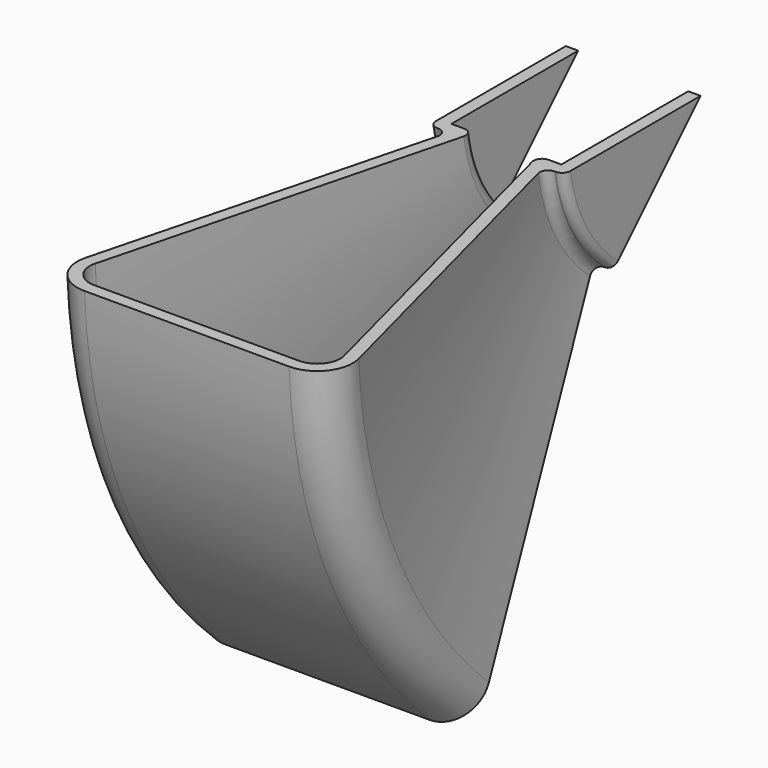
from build123d import *

# Parameters (mm, degrees)
F1_ANGLE_BACK  = 30
F1_ANGLE       = 120
F2_R           = 2
F4_DEPTH       = 25
F4_DEPTH_BACK  = 25
F5_DEPTH       = 25
F5_DEPTH_BACK  = 25
F8_R           = 5
F10_DEPTH      = 33.4248144675
F10_DEPTH_BACK = 33.4248144675
F12_DEPTH      = 50
F12_DEPTH_BACK = 50


# Not quite as in the source:
# - after a boolean that leaves OpenCascade's solid faulty, fix() repairs it
# - a feature of the source that left no trace in its solid (it failed there, or was rolled back) is left out


with BuildPart() as f1:
    # F0 (on Top) → F1 (revolve)
    with BuildSketch(Plane.XY, mode=Mode.PRIVATE) as f1_sk:
        with BuildLine():
            Line((9.6206148389, -1.9516889929), (7.6821408379, -2.0284350604))
            Line((7.6821408379, -2.0284350604), (30.2427770644, -88.5876107865))
            ThreePointArc((30.2427770644, -88.5876107865), (29.2549191731, -93.4242240292), (24.8238143675, -95.6))
            Line((24.8238143675, -95.6), (-24.8238143675, -95.6))
            ThreePointArc((-24.8238143675, -95.6), (-29.2549191731, -93.4242240292), (-30.2427770644, -88.5876107865))
            Line((-30.2427770644, -88.5876107865), (-7.6821408379, -2.0284350604))
            Line((-7.6821408379, -2.0284350604), (-9.6206148389, -1.9516889929))
            Line((-9.6206148389, -1.9516889929), (-13.35, -1.9516889929))
            Line((-13.35, -1.9516889929), (-13.35, 37))
            Line((-13.35, 37), (-16.35, 37))
            Line((-16.35, 37), (-16.35, -4.9516889929))
            Line((-16.35, -4.9516889929), (-11.5442770978, -4.9516889929))
            Line((-11.5442770978, -4.9516889929), (-33.1457927948, -87.8309737078))
            ThreePointArc((-33.1457927948, -87.8309737078), (-31.6287253189, -95.2586297591), (-24.8238143675, -98.6))
            Line((-24.8238143675, -98.6), (24.8238143675, -98.6))
            ThreePointArc((24.8238143675, -98.6), (31.6287253189, -95.2586297591), (33.1457927948, -87.8309737078))
            Line((33.1457927948, -87.8309737078), (11.5442770978, -4.9516889929))
            Line((11.5442770978, -4.9516889929), (16.35, -4.9516889929))
            Line((16.35, -4.9516889929), (16.35, 37))
            Line((16.35, 37), (13.35, 37))
            Line((13.35, 37), (13.35, -1.9516889929))
            Line((13.35, -1.9516889929), (9.6206148389, -1.9516889929))
        make_face()
    revolve(f1_sk.sketch.rotate(Axis((0.7210588083, 37, 0), (1, 0, 0)), -F1_ANGLE_BACK), axis=Axis((0.7210588083, 37, 0), (1, 0, 0)), revolution_arc=F1_ANGLE)

    # F2
    f2_edges = [f1.edges().sort_by_distance(p)[0] for p in [
        (7.682141, 3.200384, -19.514218),
        (11.544277, 0.668772, -20.975844),
        (16.35, 0.668772, -20.975844),
        (-7.682141, 3.200384, -19.514218),
        (-16.35, 0.668772, -20.975844),
        (-11.544277, 0.668772, -20.975844),
    ]]
    fillet(f2_edges, radius=F2_R)

    # F3 (on Right) → F4 (join, two sides)
    with BuildSketch(Plane.YZ) as f4_sk:
        with BuildLine():
            Line((51.55, 6), (26.6076951546, 6))
            Line((26.6076951546, 6), (34.6184301396, 1.375))
            ThreePointArc((34.6184301396, 1.375), (37.711752374, 2.6562960223), (39.75, 0))
            ThreePointArc((39.75, 0), (38.9445436483, -1.9445436483), (37, -2.75))
            Line((37, -2.75), (37, -6))
            Line((37, -6), (51.55, -6))
            Line((51.55, -6), (51.55, 6))
        make_face()
        with BuildLine():
            ThreePointArc((47.3738633754, 0.95), (47.505593785, 0.4830952573), (47.55, 0))
            ThreePointArc((47.55, 0), (47.505593785, -0.4830952573), (47.3738633754, -0.95))
            ThreePointArc((47.3738633754, -0.95), (46.7738329701, -1.8738329701), (45.85, -2.4738633754))
            ThreePointArc((45.85, -2.4738633754), (44.9, -2.65), (43.95, -2.4738633754))
            ThreePointArc((43.95, -2.4738633754), (43.0261670299, -1.8738329701), (42.4261366246, -0.95))
            ThreePointArc((42.4261366246, -0.95), (42.25, 0), (42.4261366246, 0.95))
            ThreePointArc((42.4261366246, 0.95), (43.0261670299, 1.8738329701), (43.95, 2.4738633754))
            ThreePointArc((43.95, 2.4738633754), (44.9, 2.65), (45.85, 2.4738633754))
            ThreePointArc((45.85, 2.4738633754), (46.7738329701, 1.8738329701), (47.3738633754, 0.95))
        make_face(mode=Mode.SUBTRACT)
        with BuildLine():
            Line((34.6184301396, 1.375), (26.6076951546, 6))
            Line((26.6076951546, 6), (22.45, 6))
            Line((22.45, 6), (22.45, -6))
            Line((22.45, -6), (37, -6))
            Line((37, -6), (37, -2.75))
            ThreePointArc((37, -2.75), (34.6184301396, -1.375), (34.6184301396, 1.375))
        make_face()
        with BuildLine():
            ThreePointArc((31.5738633754, 0.95), (31.705593785, 0.4830952573), (31.75, 0))
            ThreePointArc((31.75, 0), (31.705593785, -0.4830952573), (31.5738633754, -0.95))
            ThreePointArc((31.5738633754, -0.95), (30.9738329701, -1.8738329701), (30.05, -2.4738633754))
            ThreePointArc((30.05, -2.4738633754), (29.1, -2.65), (28.15, -2.4738633754))
            ThreePointArc((28.15, -2.4738633754), (27.2261670299, -1.8738329701), (26.6261366246, -0.95))
            ThreePointArc((26.6261366246, -0.95), (26.45, 0), (26.6261366246, 0.95))
            ThreePointArc((26.6261366246, 0.95), (27.2261670299, 1.8738329701), (28.15, 2.4738633754))
            ThreePointArc((28.15, 2.4738633754), (29.1, 2.65), (30.05, 2.4738633754))
            ThreePointArc((30.05, 2.4738633754), (30.9738329701, 1.8738329701), (31.5738633754, 0.95))
        make_face(mode=Mode.SUBTRACT)
        with BuildLine():
            Line((43.95, 0.95), (43.95, 2.4738633754))
            ThreePointArc((43.95, 2.4738633754), (43.0261670299, 1.8738329701), (42.4261366246, 0.95))
            Line((42.4261366246, 0.95), (43.95, 0.95))
        make_face()
        with BuildLine():
            Line((45.85, 0.95), (47.3738633754, 0.95))
            ThreePointArc((47.3738633754, 0.95), (46.7738329701, 1.8738329701), (45.85, 2.4738633754))
            Line((45.85, 2.4738633754), (45.85, 0.95))
        make_face()
        with BuildLine():
            ThreePointArc((45.85, -2.4738633754), (46.7738329701, -1.8738329701), (47.3738633754, -0.95))
            Line((47.3738633754, -0.95), (45.85, -0.95))
            Line((45.85, -0.95), (45.85, -2.4738633754))
        make_face()
        with BuildLine():
            ThreePointArc((42.4261366246, -0.95), (43.0261670299, -1.8738329701), (43.95, -2.4738633754))
            Line((43.95, -2.4738633754), (43.95, -0.95))
            Line((43.95, -0.95), (42.4261366246, -0.95))
        make_face()
        with BuildLine():
            Line((30.05, 0.95), (31.5738633754, 0.95))
            ThreePointArc((31.5738633754, 0.95), (30.9738329701, 1.8738329701), (30.05, 2.4738633754))
            Line((30.05, 2.4738633754), (30.05, 0.95))
        make_face()
        with BuildLine():
            Line((28.15, 0.95), (28.15, 2.4738633754))
            ThreePointArc((28.15, 2.4738633754), (27.2261670299, 1.8738329701), (26.6261366246, 0.95))
            Line((26.6261366246, 0.95), (28.15, 0.95))
        make_face()
        with BuildLine():
            ThreePointArc((26.6261366246, -0.95), (27.2261670299, -1.8738329701), (28.15, -2.4738633754))
            Line((28.15, -2.4738633754), (28.15, -0.95))
            Line((28.15, -0.95), (26.6261366246, -0.95))
        make_face()
        with BuildLine():
            ThreePointArc((30.05, -2.4738633754), (30.9738329701, -1.8738329701), (31.5738633754, -0.95))
            Line((31.5738633754, -0.95), (30.05, -0.95))
            Line((30.05, -0.95), (30.05, -2.4738633754))
        make_face()
    extrude(amount=F4_DEPTH)
    extrude(f4_sk.sketch, amount=-F4_DEPTH_BACK)

    # F3 (on Right) → F5 (cut, two sides)
    with BuildSketch(Plane.YZ) as f5_sk:
        with BuildLine():
            Line((37, 0), (34.6184301396, 1.375))
            ThreePointArc((34.6184301396, 1.375), (34.6184301396, -1.375), (37, -2.75))
            Line((37, -2.75), (37, 0))
        make_face()
        with BuildLine():
            ThreePointArc((31.5738633754, -0.95), (31.705593785, -0.4830952573), (31.75, 0))
            ThreePointArc((31.75, 0), (31.705593785, 0.4830952573), (31.5738633754, 0.95))
            Line((31.5738633754, 0.95), (30.05, 0.95))
            Line((30.05, 0.95), (30.05, 2.4738633754))
            ThreePointArc((30.05, 2.4738633754), (29.1, 2.65), (28.15, 2.4738633754))
            Line((28.15, 2.4738633754), (28.15, 0.95))
            Line((28.15, 0.95), (26.6261366246, 0.95))
            ThreePointArc((26.6261366246, 0.95), (26.45, 0), (26.6261366246, -0.95))
            Line((26.6261366246, -0.95), (28.15, -0.95))
            Line((28.15, -0.95), (28.15, -2.4738633754))
            ThreePointArc((28.15, -2.4738633754), (29.1, -2.65), (30.05, -2.4738633754))
            Line((30.05, -2.4738633754), (30.05, -0.95))
            Line((30.05, -0.95), (31.5738633754, -0.95))
        make_face()
    extrude(amount=-F5_DEPTH, mode=Mode.SUBTRACT)
    extrude(f5_sk.sketch, amount=F5_DEPTH_BACK, mode=Mode.SUBTRACT)

    add(f1.part.fix(), mode=Mode.REPLACE)

    # F8
    f8_edges = [f1.edges().sort_by_distance(p)[0] for p in [
        (-20.675, 22.45, -6),
        (-20.675, 22.45, 6),
        (0, 51.55, 6),
        (0, 51.55, -6),
    ]]
    fillet(f8_edges, radius=F8_R)

    # F9 (on Right) → F10 (cut, two sides)
    with BuildSketch(Plane.YZ) as f10_sk:
        Polygon((-115.0443181396, -6), (27.45, -6), (46.55, -6), (89.7687226534, -48.6618503928), (83.2566171885, 31.4302965999), (-50.0242002308, 71.4145377278), (-90.0084450841, 71.4145377278), align=None)
    extrude(amount=F10_DEPTH, mode=Mode.SUBTRACT)
    extrude(f10_sk.sketch, amount=-F10_DEPTH_BACK, mode=Mode.SUBTRACT)

    # F11 (on Right) → F12 (cut, two sides)
    with BuildSketch(Plane.YZ) as f12_sk:
        Polygon((57.0278279483, 8.6879674345), (37, -6), (-77.3825557827, -120.3825557827), (-35.5902947485, -136.9153559208), (64.6576955914, -143.4855163097), (76.9502595067, -111.2705171108), (76.9502595067, -24.7986763716), align=None)
    extrude(amount=-F12_DEPTH, mode=Mode.SUBTRACT)
    extrude(f12_sk.sketch, amount=F12_DEPTH_BACK, mode=Mode.SUBTRACT)


solid = f1.part
